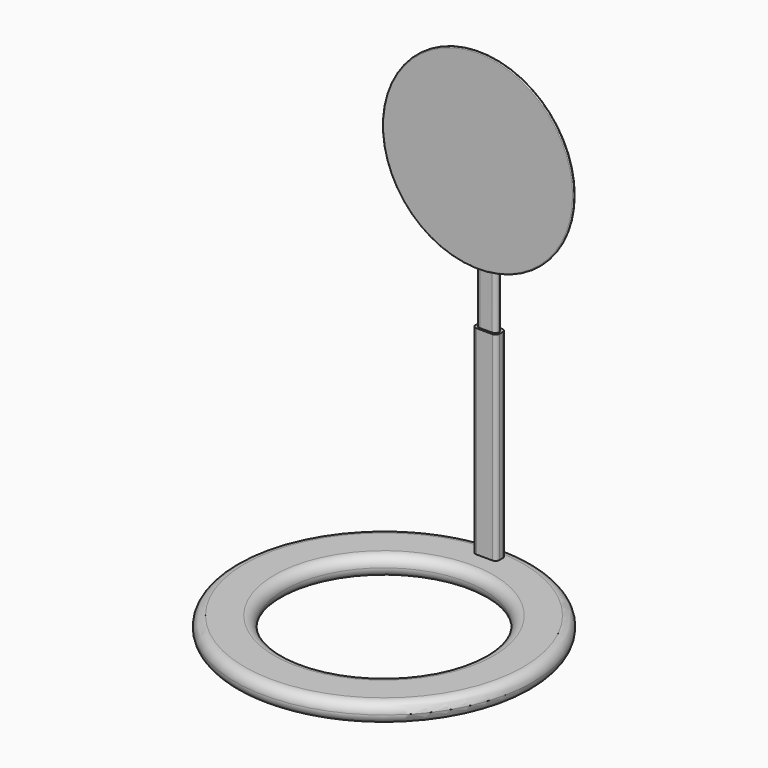
from build123d import *

# Parameters (mm, degrees)
F0_R      = 75
F0_R_2    = 50
F1_DEPTH  = 10
F2_R      = 4.99999
F3_W      = 12
F3_H      = 6
F4_DEPTH  = 100
F5_R      = 2
F6_W      = 10
F6_H      = 4
F7_DEPTH  = 90
F8_R      = 1.99999
F10_DEPTH = 1
F11_R     = 6
F12_DEPTH = 1
F13_R     = 12
F14_DEPTH = 1
F15_R     = 24
F16_DEPTH = 1
F17_R     = 48
F18_DEPTH = 1
F19_R     = 0.49999


# Not quite as in the source:
# - a fillet or chamfer is up to 0.001 mm smaller than in the source, because OpenCascade refuses the exact size


with BuildPart() as f1:
    # F0 (on Top) → F1 (new body)
    with BuildSketch(Plane.XY):
        Circle(F0_R)
        Circle(F0_R_2, mode=Mode.SUBTRACT)
    extrude(amount=F1_DEPTH)

    # F2 (radius 5 in the source; OpenCascade refuses exactly that, so slightly less here)
    f2_edges = [f1.edges().sort_by_distance(p)[0] for p in [
        (-75, 0, 10),
        (-50, 0, 10),
        (-75, 0, 0),
        (-50, 0, 0),
    ]]
    fillet(f2_edges, radius=F2_R)

    # F3 (on face) → F4 (join)
    with BuildSketch(Plane.XY.offset(10)):
        with Locations((0, 66)):
            Rectangle(F3_W, F3_H)
    extrude(amount=F4_DEPTH)

    # F5
    f5_edges = [f1.edges().sort_by_distance(p)[0] for p in [
        (6, 69, 60),
        (6, 63, 60),
        (-6, 69, 60),
        (-6, 63, 60),
    ]]
    fillet(f5_edges, radius=F5_R)

    # F6 (on face) → F7 (join)
    with BuildSketch(Plane.XY.offset(110)):
        with Locations((0, 66)):
            Rectangle(F6_W, F6_H)
    extrude(amount=F7_DEPTH)

    # F8 (radius 2 in the source; OpenCascade refuses exactly that, so slightly less here)
    f8_edges = [f1.edges().sort_by_distance(p)[0] for p in [
        (5, 64, 155),
        (5, 68, 155),
        (-5, 68, 155),
        (-5, 64, 155),
        (-5, 66, 200),
        (5, 66, 200),
        (0, 68, 200),
        (0, 64, 200),
    ]]
    fillet(f8_edges, radius=F8_R)


with BuildPart() as f10:
    # F9 (on face) → F10 (new body)
    with BuildSketch(Plane.XZ.offset(-64)):
        with BuildLine():
            ThreePointArc((-3, 186.9557797909), (0, 183.9557797909), (3, 186.9557797909))
            ThreePointArc((3, 186.9557797909), (0, 189.9557797909), (-3, 186.9557797909))
        make_face()
    extrude(amount=F10_DEPTH)

    # F11 (on face) → F12 (join)
    with BuildSketch(Plane.XZ.offset(-63)):
        with Locations((0, 186.9557797909)):
            Circle(F11_R)
    extrude(amount=F12_DEPTH)

    # F13 (on face) → F14 (join)
    with BuildSketch(Plane.XZ.offset(-62)):
        with Locations((0, 186.9557797909)):
            Circle(F13_R)
    extrude(amount=F14_DEPTH)

    # F15 (on face) → F16 (join)
    with BuildSketch(Plane.XZ.offset(-61)):
        with Locations((0, 186.9557797909)):
            Circle(F15_R)
    extrude(amount=F16_DEPTH)

    # F17 (on face) → F18 (join)
    with BuildSketch(Plane.XZ.offset(-60)):
        with Locations((0, 186.9557797909)):
            Circle(F17_R)
    extrude(amount=F18_DEPTH)

    # F19 (radius 0.5 in the source; OpenCascade refuses exactly that, so slightly less here)
    f19_edges = [f10.edges().sort_by_distance(p)[0] for p in [
        (-48, 59, 186.95578),
        (-48, 60, 186.95578),
        (-24, 60, 186.95578),
        (-24, 61, 186.95578),
        (-12, 61, 186.95578),
        (-12, 62, 186.95578),
        (-6, 62, 186.95578),
        (-6, 63, 186.95578),
        (3, 63, 186.95578),
        (3, 64, 186.95578),
    ]]
    fillet(f19_edges, radius=F19_R)


solid = Compound([f1.part, f10.part])
